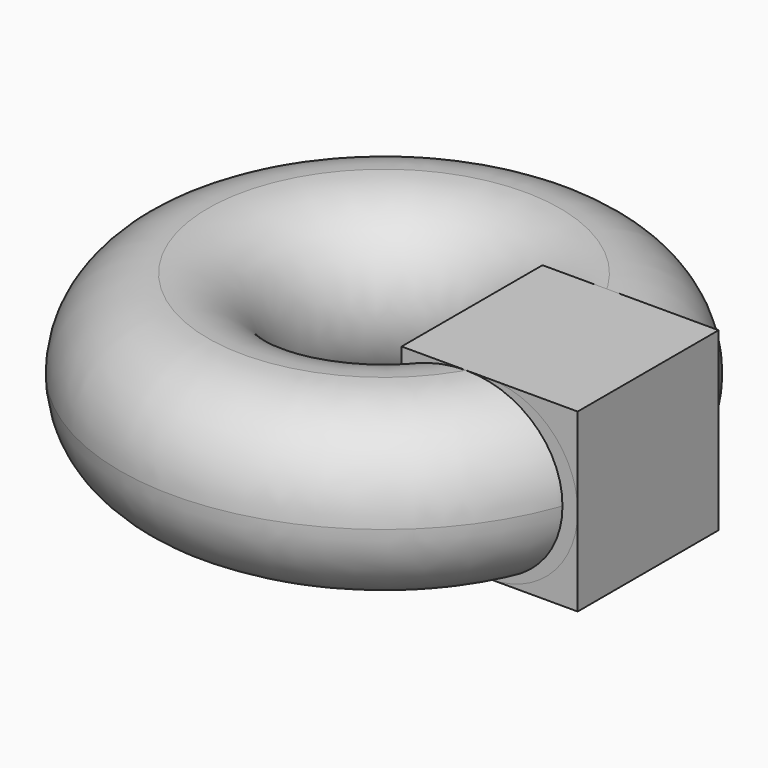
from build123d import *

# Parameters (mm, degrees)
F0_W     = 100
F0_H     = 100
F1_DEPTH = 50
F3_DEPTH = 50


with BuildPart() as f1:
    # F0 (on Front) → F1 (new body, symmetric)
    with BuildSketch(Plane.XZ):
        Rectangle(F0_W, F0_H)
    extrude(amount=F1_DEPTH, both=True)


with BuildPart() as f3:
    # F2 (on Front) → F3 (new body, symmetric)
    with BuildSketch(Plane.XZ):
        with BuildLine():
            Line((0, -50), (0, 50))
            ThreePointArc((0, 50), (-50, 0), (0, -50))
        make_face()
        with BuildLine():
            ThreePointArc((0, -50), (35.355339, -35.355339), (50, 0))
            ThreePointArc((50, 0), (35.355339, 35.355339), (0, 50))
            Line((0, 50), (0, -50))
        make_face()
    extrude(amount=F3_DEPTH, both=True)


with BuildPart() as f4:
    # F2 (on Front) → F4 (revolve)
    with BuildSketch(Plane.XZ):
        with BuildLine():
            Line((0, -50), (0, 50))
            ThreePointArc((0, 50), (-50, 0), (0, -50))
        make_face()
    revolve(axis=Axis((0, 0, 0), (0, 0, -1)))


with BuildPart() as f5:
    # F2 (on Front) → F5 (revolve)
    with BuildSketch(Plane.XZ):
        with BuildLine():
            ThreePointArc((0, -50), (35.355339, -35.355339), (50, 0))
            ThreePointArc((50, 0), (35.355339, 35.355339), (0, 50))
            Line((0, 50), (0, -50))
        make_face()
        with BuildLine():
            Line((0, -50), (0, 50))
            ThreePointArc((0, 50), (-50, 0), (0, -50))
        make_face()
    revolve(axis=Axis((-100, 0, 0), (0, 0, -1)))


with BuildPart() as f6:
    # F2 (on Front) → F6 (revolve)
    with BuildSketch(Plane.XZ):
        with BuildLine():
            Line((0, -50), (0, 50))
            ThreePointArc((0, 50), (-50, 0), (0, -50))
        make_face()
    revolve(axis=Axis((-100, 0, 0), (0, 0, -1)))


solid = Compound([f1.part, f3.part, f4.part, f5.part, f6.part])
